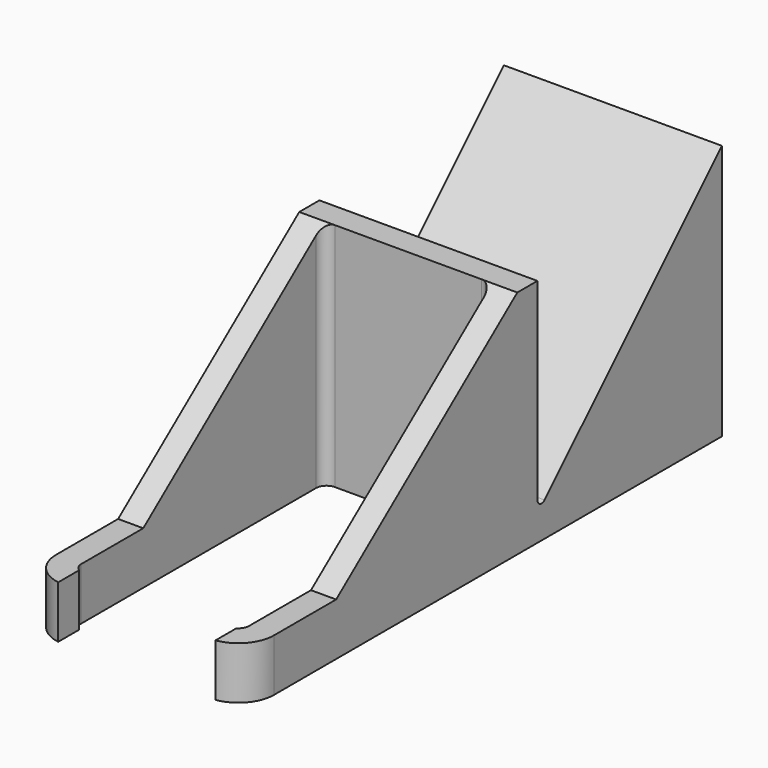
from build123d import *

# Parameters (mm, degrees)
F6_DEPTH       = 10.4
F8_DEPTH       = 22
F9_W           = 15
F9_H           = 3.4
F10_DEPTH      = 24.401
F12_DEPTH      = 10.401
F12_DEPTH_BACK = 10.401
F14_DEPTH      = 8


with BuildPart() as f6:
    # F5 (on Right) → F6 (new body, symmetric)
    with BuildSketch(Plane.YZ):
        with BuildLine():
            Line((24.4, 0), (24.4, 24.4))
            Line((24.4, 24.4), (3.2535533906, 3.2535533906))
            ThreePointArc((3.2535533906, 3.2535533906), (2.7086582838, 3.1451670149), (2.4, 3.6071067812))
            Line((2.4, 3.6071067812), (2.4, 22))
            Line((2.4, 22), (0, 22))
            Line((0, 22), (0, 0))
            Line((0, 0), (24.4, 0))
        make_face()
    extrude(amount=F6_DEPTH, both=True)

    # F7 (on Top) → F8 (join)
    with BuildSketch(Plane.XY):
        with BuildLine():
            Line((-7, 0), (-10.4, 0))
            Line((-10.4, 0), (-10.4, -21.6))
            Line((-10.4, -21.6), (-10.4, -29))
            ThreePointArc((-10.4, -29), (-9.404163056, -31.404163056), (-7, -32.4))
            Line((-7, -32.4), (7, -32.4))
            ThreePointArc((7, -32.4), (9.404163056, -31.404163056), (10.4, -29))
            Line((10.4, -29), (10.4, -21.6))
            Line((10.4, -21.6), (10.4, 0))
            Line((10.4, 0), (7, 0))
            ThreePointArc((7, 0), (7.7071067812, -0.2928932188), (8, -1))
            Line((8, -1), (8, -29))
            ThreePointArc((8, -29), (7.7071067812, -29.7071067812), (7, -30))
            Line((7, -30), (-7, -30))
            ThreePointArc((-7, -30), (-7.7071067812, -29.7071067812), (-8, -29))
            Line((-8, -29), (-8, -1))
            ThreePointArc((-8, -1), (-7.7071067812, -0.2928932188), (-7, 0))
        make_face()
    extrude(amount=F8_DEPTH)

    # F9 (on Top) → F10 (cut, through all)
    with BuildSketch(Plane.XY):
        with Locations((0, -30.7)):
            Rectangle(F9_W, F9_H)
    extrude(amount=F10_DEPTH, mode=Mode.SUBTRACT)

    # F11 (on Right) → F12 (cut, two sides)
    with BuildSketch(Plane.YZ) as f12_sk:
        Polygon((-32.4, 22), (-32.4, 5), (-21.6, 5), (0, 22), align=None)
    extrude(amount=F12_DEPTH, mode=Mode.SUBTRACT)
    extrude(f12_sk.sketch, amount=-F12_DEPTH_BACK, mode=Mode.SUBTRACT)

    # F13 (on Right) → F14 (cut, symmetric)
    with BuildSketch(Plane.YZ):
        Polygon((24.4, 2.4), (24.4, 21.0058874503), (5.7941125497, 2.4), align=None)
    extrude(amount=F14_DEPTH, both=True, mode=Mode.SUBTRACT)


solid = f6.part
